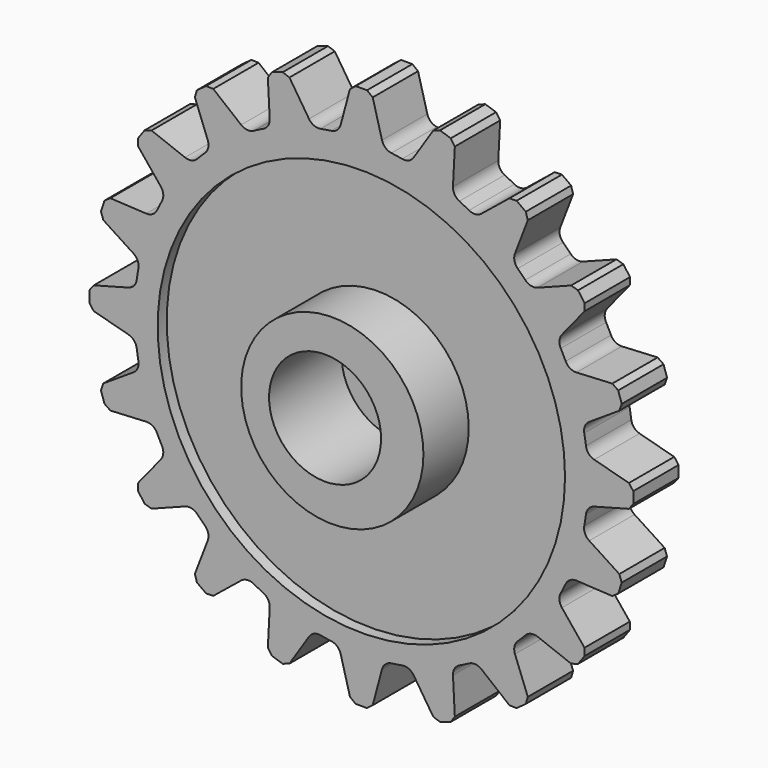
from build123d import *

# Parameters (mm, degrees)
F0_R            = 100
F1_DEPTH        = 25
F3_DEPTH        = 25
F3_COPIES_COUNT = 20
F4_SIZE         = 2
F5_R            = 5
F6_R            = 89.8821590501
F7_DEPTH        = 5
F8_R            = 40.2102253777
F9_DEPTH        = 25
F10_R           = 24.7131029744
F11_DEPTH       = 15
F12_DEPTH       = 25


# Not quite as in the source:
# - a pattern or mirror of a feature is missing from the dataset's text; its kind, count and spacing are read off the source's solid


with BuildPart() as f1:
    # F0 (on Front) → F1 (new body)
    with BuildSketch(Plane.XZ):
        Circle(F0_R)
    extrude(amount=F1_DEPTH)

    # F2 (on Front) → F3 (join)
    with BuildSketch(Plane.XZ):
        Polygon((-4.5, 120), (-9.9931095726, 99.4994359837), (9.9931095726, 99.4994359837), (4.5, 120), align=None)
    f3 = extrude(amount=F3_DEPTH)

    # F3_copies: F3 ×20 about axis
    f3_copies_axis = Axis((0, 0, 0), (0, 1, 0))
    for i in range(1, F3_COPIES_COUNT):
        add(f3.rotate(f3_copies_axis, i * 360 / F3_COPIES_COUNT))

    # F4
    f4_edges = [f1.edges().sort_by_distance(p)[0] for p in [
        (4.5, -12.5, 120),
        (-4.5, -12.5, 120),
        (-32.802285, -12.5, 115.517358),
        (115.517358, -12.5, 32.802285),
        (120, -12.5, 4.5),
        (120, -12.5, -4.5),
        (115.517358, -12.5, -32.802285),
        (112.736205, -12.5, -41.361794),
        (99.727073, -12.5, -66.893654),
        (94.437006, -12.5, -74.174807),
        (74.174807, -12.5, -94.437006),
        (66.893654, -12.5, -99.727073),
        (41.361794, -12.5, -112.736205),
        (32.802285, -12.5, -115.517358),
        (4.5, -12.5, -120),
        (-4.5, -12.5, -120),
        (-32.802285, -12.5, -115.517358),
        (-41.361794, -12.5, -112.736205),
        (-66.893654, -12.5, -99.727073),
        (-74.174807, -12.5, -94.437006),
        (-94.437006, -12.5, -74.174807),
        (-99.727073, -12.5, -66.893654),
        (-112.736205, -12.5, -41.361794),
        (-115.517358, -12.5, -32.802285),
        (-120, -12.5, -4.5),
        (-120, -12.5, 4.5),
        (-115.517358, -12.5, 32.802285),
        (-112.736205, -12.5, 41.361794),
        (-99.727073, -12.5, 66.893654),
        (-94.437006, -12.5, 74.174807),
        (-74.174807, -12.5, 94.437006),
        (-66.893654, -12.5, 99.727073),
        (32.802285, -12.5, 115.517358),
        (41.361794, -12.5, 112.736205),
        (66.893654, -12.5, 99.727073),
        (74.174807, -12.5, 94.437006),
        (94.437006, -12.5, 74.174807),
        (99.727073, -12.5, 66.893654),
        (112.736205, -12.5, 41.361794),
        (-41.361794, -12.5, 112.736205),
    ]]
    chamfer(f4_edges, length=F4_SIZE)

    # F5
    f5_edges = [f1.edges().sort_by_distance(p)[0] for p in [
        (9.99311, -12.5, 99.499436),
        (-9.99311, -12.5, 99.499436),
        (97.717628, -12.5, 21.243005),
        (99.499436, -12.5, 9.99311),
        (91.541546, -12.5, 40.251029),
        (86.370537, -12.5, 50.399706),
        (99.499436, -12.5, -9.99311),
        (97.717628, -12.5, -21.243005),
        (74.622932, -12.5, 66.568897),
        (66.568897, -12.5, 74.622932),
        (91.541546, -12.5, -40.251029),
        (86.370537, -12.5, -50.399706),
        (50.399706, -12.5, 86.370537),
        (40.251029, -12.5, 91.541546),
        (74.622932, -12.5, -66.568897),
        (66.568897, -12.5, -74.622932),
        (21.243005, -12.5, 97.717628),
        (50.399706, -12.5, -86.370537),
        (40.251029, -12.5, -91.541546),
        (-21.243005, -12.5, 97.717628),
        (21.243005, -12.5, -97.717628),
        (9.99311, -12.5, -99.499436),
        (-40.251029, -12.5, 91.541546),
        (-50.399706, -12.5, 86.370537),
        (-9.99311, -12.5, -99.499436),
        (-21.243005, -12.5, -97.717628),
        (-66.568897, -12.5, 74.622932),
        (-74.622932, -12.5, 66.568897),
        (-40.251029, -12.5, -91.541546),
        (-50.399706, -12.5, -86.370537),
        (-86.370537, -12.5, 50.399706),
        (-91.541546, -12.5, 40.251029),
        (-66.568897, -12.5, -74.622932),
        (-74.622932, -12.5, -66.568897),
        (-97.717628, -12.5, 21.243005),
        (-99.499436, -12.5, 9.99311),
        (-86.370537, -12.5, -50.399706),
        (-91.541546, -12.5, -40.251029),
        (-99.499436, -12.5, -9.99311),
        (-97.717628, -12.5, -21.243005),
    ]]
    fillet(f5_edges, radius=F5_R)

    # F6 (on face) → F7 (cut)
    with BuildSketch(Plane.XZ.offset(25)):
        with Locations((0, -1.6950928839)):
            Circle(F6_R)
    extrude(amount=-F7_DEPTH, mode=Mode.SUBTRACT)

    # F8 (on face) → F9 (join)
    with BuildSketch(Plane.XZ.offset(20)):
        with Locations((3.1838121358, 0)):
            Circle(F8_R)
    extrude(amount=F9_DEPTH)

    # F10 (on face) → F11 (cut)
    with BuildSketch(Plane.XZ.offset(45)):
        Circle(F10_R)
    extrude(amount=-F11_DEPTH, mode=Mode.SUBTRACT)

    # F12 (cut): a face of the model
    f12_faces = [f1.faces().sort_by_distance(p)[0] for p in [
        (0, -30, 0),
    ]]
    extrude(f12_faces, amount=-F12_DEPTH, mode=Mode.SUBTRACT)


solid = f1.part
